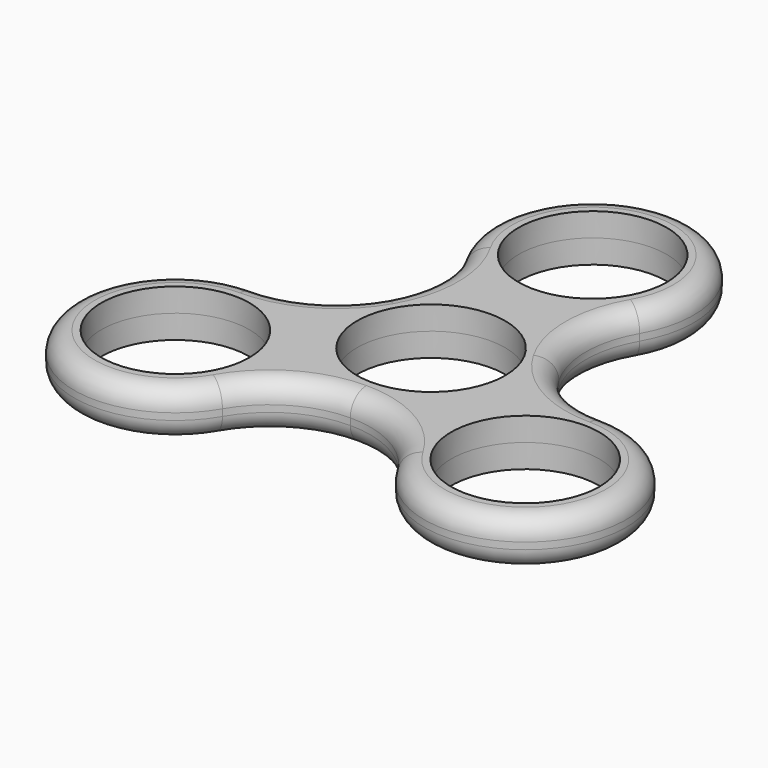
from build123d import *

# Parameters (mm, degrees)
F0_R     = 11
F1_DEPTH = 3.5
F2_R     = 3
F3_R     = 3


# Not quite as in the source:
# - a feature names something its author has since deleted; it is built from what else it names


with BuildPart() as f1:
    # F0 (on Top) → F1 (new body, symmetric)
    with BuildSketch(Plane.XY):
        with BuildLine():
            ThreePointArc((0, 15), (7.4999998929, 12.9903811186), (12.990380933, 7.5000002143))
            ThreePointArc((12.990380933, 7.5000002143), (10.9807621135, 15.0000001237), (12.9903810568, 22.5))
            ThreePointArc((12.9903810568, 22.5), (7.5, 17.0096189432), (0, 15))
        make_face()
        with BuildLine():
            ThreePointArc((-12.9903810309, 7.5000000448), (-7.4999999776, 12.9903810697), (0, 15))
            ThreePointArc((0, 15), (-7.5, 17.0096189432), (-12.9903810568, 22.5))
            ThreePointArc((-12.9903810568, 22.5), (-10.9807621135, 15.0000000259), (-12.9903810309, 7.5000000448))
        make_face()
        with BuildLine():
            ThreePointArc((-12.9903810914, -7.49999994), (-15, 6.05e-08), (-12.9903810309, 7.5000000448))
            ThreePointArc((-12.9903810309, 7.5000000448), (-18.4807620911, 2.0096189562), (-25.9807621135, 0))
            ThreePointArc((-25.9807621135, 0), (-18.4807621435, -2.0096189259), (-12.9903810914, -7.49999994))
        make_face()
        with BuildLine():
            ThreePointArc((-12.9903810568, -22.5), (-7.5, -17.0096189433), (-1e-10, -15))
            ThreePointArc((-1e-10, -15), (-7.50000003, -12.9903810394), (-12.9903810914, -7.49999994))
            ThreePointArc((-12.9903810914, -7.49999994), (-11.4918747282, -11.11771429), (-10.9807621135, -15))
            ThreePointArc((-10.9807621135, -15), (-11.4918747192, -18.8822856765), (-12.9903810568, -22.5))
        make_face()
        with BuildLine():
            ThreePointArc((12.9903810568, -22.5), (10.9807621135, -15.0000001847), (12.9903808721, -7.5000003199))
            ThreePointArc((12.9903808721, -7.5000003199), (7.49999984, -12.9903811491), (-1e-10, -15))
            ThreePointArc((-1e-10, -15), (7.5, -17.0096189432), (12.9903810568, -22.5))
        make_face()
        with BuildLine():
            ThreePointArc((12.990380933, 7.5000002143), (14.4888873623, 3.882285796), (15, 0))
            ThreePointArc((15, 0), (14.4888873465, -3.882285855), (12.9903808721, -7.5000003199))
            ThreePointArc((12.9903808721, -7.5000003199), (18.4807619536, -2.0096190356), (25.9807621135, 0))
            ThreePointArc((25.9807621135, 0), (18.4807620064, 2.0096190051), (12.990380933, 7.5000002143))
        make_face()
        with BuildLine():
            ThreePointArc((12.9903808721, -7.5000003199), (14.4888873465, -3.882285855), (15, 0))
            ThreePointArc((15, 0), (14.4888873623, 3.882285796), (12.990380933, 7.5000002143))
            ThreePointArc((12.990380933, 7.5000002143), (7.4999998929, 12.9903811186), (0, 15))
            ThreePointArc((0, 15), (-7.4999999776, 12.9903810697), (-12.9903810309, 7.5000000448))
            ThreePointArc((-12.9903810309, 7.5000000448), (-15, 6.05e-08), (-12.9903810914, -7.49999994))
            ThreePointArc((-12.9903810914, -7.49999994), (-7.50000003, -12.9903810394), (-1e-10, -15))
            ThreePointArc((-1e-10, -15), (7.49999984, -12.9903811491), (12.9903808721, -7.5000003199))
        make_face()
        Circle(F0_R, mode=Mode.SUBTRACT)
        with BuildLine():
            ThreePointArc((-12.9903810568, 22.5), (-7.5, 17.0096189432), (0, 15))
            ThreePointArc((0, 15), (7.5, 17.0096189432), (12.9903810568, 22.5))
            ThreePointArc((12.9903810568, 22.5), (14.4888873943, 26.1177143235), (15, 30))
            ThreePointArc((15, 30), (-3.8822856765, 44.4888873943), (-12.9903810568, 22.5))
        make_face()
        with Locations((0, 30)):
            Circle(F0_R, mode=Mode.SUBTRACT)
        with BuildLine():
            ThreePointArc((25.9807621135, 0), (18.4807619536, -2.0096190356), (12.9903808721, -7.5000003199))
            ThreePointArc((12.9903808721, -7.5000003199), (10.9807621135, -15.0000001847), (12.9903810568, -22.5))
            ThreePointArc((12.9903810568, -22.5), (29.8630477901, -29.4888873943), (40.9807621135, -15))
            ThreePointArc((40.9807621135, -15), (36.5873638313, -4.3933982822), (25.9807621135, 0))
        make_face()
        with Locations((25.9807621135, -15)):
            Circle(F0_R, mode=Mode.SUBTRACT)
        with BuildLine():
            ThreePointArc((-10.9807621135, -15), (-11.4918747282, -11.11771429), (-12.9903810914, -7.49999994))
            ThreePointArc((-12.9903810914, -7.49999994), (-18.4807621435, -2.0096189259), (-25.9807621135, 0))
            ThreePointArc((-25.9807621135, 0), (-38.9711431703, -22.5), (-12.9903810568, -22.5))
            ThreePointArc((-12.9903810568, -22.5), (-11.4918747192, -18.8822856765), (-10.9807621135, -15))
        make_face()
        with Locations((-25.9807621135, -15)):
            Circle(F0_R, mode=Mode.SUBTRACT)
    extrude(amount=F1_DEPTH, both=True)

    # F2
    f2_edges = [f1.edges().sort_by_distance(p)[0] for p in [
        (38.971143, -22.5, 3.5),
    ]]
    fillet(f2_edges, radius=F2_R)

    # F3
    f3_edges = [f1.edges().sort_by_distance(p)[0] for p in [
        (0, -15, -3.5),
    ]]
    fillet(f3_edges, radius=F3_R)


solid = f1.part
